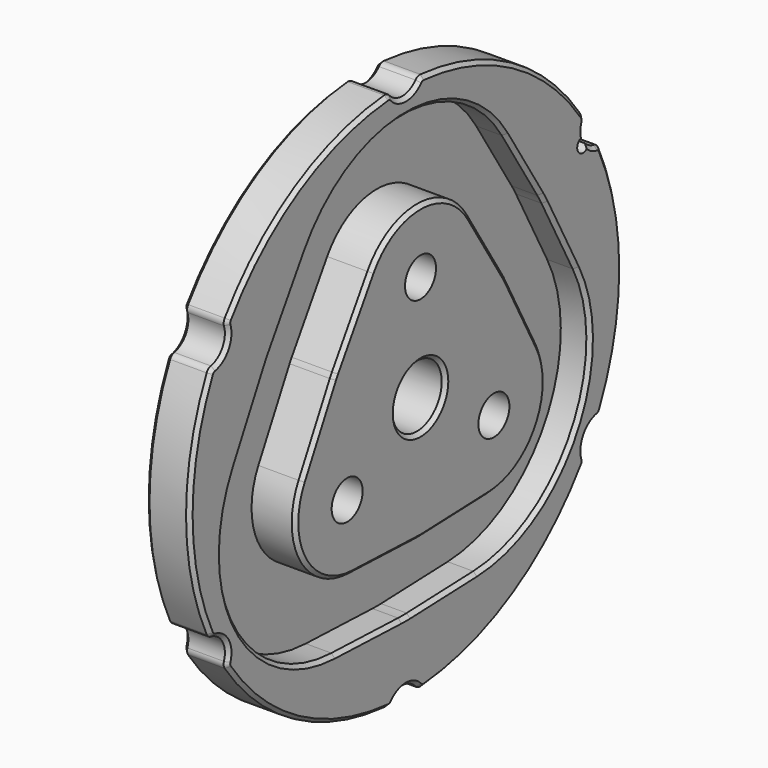
from build123d import *

# Parameters (mm, degrees)
F0_R     = 2.65
F0_R_2   = 4.25
F1_DEPTH = 6
F2_DEPTH = 4
F3_DEPTH = 2
F4_SIZE  = 0.5
F5_SIZE2 = 2.3
F5_SIZE  = 5


# Not quite as in the source:
# - two fillets or chamfers of one size are made in one step


with BuildPart() as f1:
    # F0 (on Right) → F1 (new body)
    with BuildSketch(Plane.YZ):
        with BuildLine():
            ThreePointArc((-2.2515407231, 36.53242851), (-2.6294191421, 36.8013801393), (-3.0879953604, 36.8709138028))
            ThreePointArc((-3.0879953604, 36.8709138028), (-18.5, 32.04293994), (-30.3871503338, 21.1097393303))
            ThreePointArc((-30.3871503338, 21.1097393303), (-30.5562205239, 20.6778338439), (-30.5122407901, 20.2161057189))
            ThreePointArc((-30.5122407901, 20.2161057189), (-30.7524645978, 17.7549437138), (-32.7637815132, 16.3163227911))
            ThreePointArc((-32.7637815132, 16.3163227911), (-33.185639666, 16.1235462954), (-33.4751456942, 15.7611744725))
            ThreePointArc((-33.4751456942, 15.7611744725), (-37, 0), (-33.4751456942, -15.7611744725))
            ThreePointArc((-33.4751456942, -15.7611744725), (-33.185639666, -16.1235462954), (-32.7637815132, -16.3163227911))
            ThreePointArc((-32.7637815132, -16.3163227911), (-30.7524645978, -17.7549437138), (-30.5122407901, -20.2161057189))
            ThreePointArc((-30.5122407901, -20.2161057189), (-30.5562205239, -20.6778338439), (-30.3871503338, -21.1097393303))
            ThreePointArc((-30.3871503338, -21.1097393303), (-18.5, -32.04293994), (-3.0879953604, -36.8709138028))
            ThreePointArc((-3.0879953604, -36.8709138028), (-2.6294191421, -36.8013801393), (-2.2515407231, -36.53242851))
            ThreePointArc((-2.2515407231, -36.53242851), (0, -35.5098874275), (2.2515407231, -36.53242851))
            ThreePointArc((2.2515407231, -36.53242851), (2.6294191421, -36.8013801393), (3.0879953604, -36.8709138028))
            ThreePointArc((3.0879953604, -36.8709138028), (18.5, -32.04293994), (30.3871503338, -21.1097393303))
            ThreePointArc((30.3871503338, -21.1097393303), (30.5562205239, -20.6778338439), (30.5122407901, -20.2161057189))
            ThreePointArc((30.5122407901, -20.2161057189), (30.7524645978, -17.7549437138), (32.7637815132, -16.3163227911))
            ThreePointArc((32.7637815132, -16.3163227911), (33.185639666, -16.1235462954), (33.4751456942, -15.7611744725))
            ThreePointArc((33.4751456942, -15.7611744725), (37, 0), (33.4751456942, 15.7611744725))
            ThreePointArc((33.4751456942, 15.7611744725), (33.185639666, 16.1235462954), (32.7637815132, 16.3163227911))
            ThreePointArc((32.7637815132, 16.3163227911), (31.941237039, 16.6082774884), (31.2380455813, 17.1253255822))
            ThreePointArc((31.2380455813, 17.1253255822), (29.4448637287, 17), (30.449989793, 18.4902782469))
            ThreePointArc((30.449989793, 18.4902782469), (30.3538087376, 19.3577839598), (30.5122407901, 20.2161057189))
            ThreePointArc((30.5122407901, 20.2161057189), (30.5562205239, 20.6778338439), (30.3871503338, 21.1097393303))
            ThreePointArc((30.3871503338, 21.1097393303), (18.5, 32.04293994), (3.0879953604, 36.8709138028))
            ThreePointArc((3.0879953604, 36.8709138028), (2.6294191421, 36.8013801393), (2.2515407231, 36.53242851))
            ThreePointArc((2.2515407231, 36.53242851), (0, 35.5098874275), (-2.2515407231, 36.53242851))
        make_face()
        with BuildLine():
            Line((-23.0952370323, 14.180454946), (-17.0328632471, 23.8484731203))
            ThreePointArc((-17.0328632471, 23.8484731203), (0.0002590164, 33.2703478915), (17.0295377344, 23.8415279974))
            Line((17.0295377344, 23.8415279974), (23.0899184639, 14.167925942))
            ThreePointArc((23.0899184639, 14.167925942), (23.4636524397, 13.5467460522), (23.8147430167, 12.9124929901))
            Line((23.8147430167, 12.9124929901), (29.162137778, 2.827248294))
            ThreePointArc((29.162137778, 2.827248294), (28.813095975, -16.6349496309), (12.1369519401, -26.6751288313))
            Line((12.1369519401, -26.6751288313), (0.7330157043, -27.0912894495))
            ThreePointArc((0.7330157043, -27.0912894495), (0, -27.1046598669), (-0.7330157043, -27.0912894495))
            Line((-0.7330157043, -27.0912894495), (-12.1441739659, -26.6748652799))
            ThreePointArc((-12.1441739659, -26.6748652799), (-28.8182692269, -16.6382354957), (-29.1731979579, 2.8202694775))
            Line((-29.1731979579, 2.8202694775), (-23.8282527367, 12.9108345034))
            ThreePointArc((-23.8282527367, 12.9108345034), (-23.4733240056, 13.5523299334), (-23.0952370323, 14.180454946))
        make_face(mode=Mode.SUBTRACT)
        with BuildLine():
            ThreePointArc((17.0295377344, 23.8415279974), (0.0002590164, 33.2703478915), (-17.0328632471, 23.8484731203))
            Line((-17.0328632471, 23.8484731203), (-23.0952370323, 14.180454946))
            ThreePointArc((-23.0952370323, 14.180454946), (-23.4733240056, 13.5523299334), (-23.8282527367, 12.9108345034))
            Line((-23.8282527367, 12.9108345034), (-29.1731979579, 2.8202694775))
            ThreePointArc((-29.1731979579, 2.8202694775), (-28.8182692269, -16.6382354957), (-12.1441739659, -26.6748652799))
            Line((-12.1441739659, -26.6748652799), (-0.7330157043, -27.0912894495))
            ThreePointArc((-0.7330157043, -27.0912894495), (0, -27.1046598669), (0.7330157043, -27.0912894495))
            Line((0.7330157043, -27.0912894495), (12.1369519401, -26.6751288313))
            ThreePointArc((12.1369519401, -26.6751288313), (28.813095975, -16.6349496309), (29.162137778, 2.827248294))
            Line((29.162137778, 2.827248294), (23.8147430167, 12.9124929901))
            ThreePointArc((23.8147430167, 12.9124929901), (23.4636524397, 13.5467460522), (23.0899184639, 14.167925942))
            Line((23.0899184639, 14.167925942), (17.0295377344, 23.8415279974))
        make_face()
        with BuildLine():
            Line((-14.5383641102, 8.8148297318), (-8.4759903249, 18.482847906))
            ThreePointArc((-8.4759903249, 18.482847906), (-0.0018003141, 23.1703476982), (8.4704774851, 18.4793926211))
            Line((8.4704774851, 18.4793926211), (14.5308582146, 8.8057905657))
            ThreePointArc((14.5308582146, 8.8057905657), (14.7167955123, 8.4967458506), (14.8914674376, 8.1811970698))
            Line((14.8914674376, 8.1811970698), (20.2388621989, -1.9040476263))
            ThreePointArc((20.2388621989, -1.9040476263), (20.0652095641, -11.5867329668), (11.7686206585, -16.5818468966))
            Line((11.7686206585, -16.5818468966), (0.3646844227, -16.9980075148))
            ThreePointArc((0.3646844227, -16.9980075148), (0, -17.0046594636), (-0.3646844227, -16.9980075148))
            Line((-0.3646844227, -16.9980075148), (-11.7758426843, -16.5815833453))
            ThreePointArc((-11.7758426843, -16.5815833453), (-20.0714122995, -11.5882352941), (-20.2479937541, -1.9073872429))
            Line((-20.2479937541, -1.9073872429), (-14.9030485329, 8.183177783))
            ThreePointArc((-14.9030485329, 8.183177783), (-14.7264670782, 8.5023297318), (-14.5383641102, 8.8148297318))
        make_face(mode=Mode.SUBTRACT)
        with BuildLine():
            ThreePointArc((8.4704774851, 18.4793926211), (-0.0018003141, 23.1703476982), (-8.4759903249, 18.482847906))
            Line((-8.4759903249, 18.482847906), (-14.5383641102, 8.8148297318))
            ThreePointArc((-14.5383641102, 8.8148297318), (-14.7264670782, 8.5023297318), (-14.9030485329, 8.183177783))
            Line((-14.9030485329, 8.183177783), (-20.2479937541, -1.9073872429))
            ThreePointArc((-20.2479937541, -1.9073872429), (-20.0714122995, -11.5882352941), (-11.7758426843, -16.5815833453))
            Line((-11.7758426843, -16.5815833453), (-0.3646844227, -16.9980075148))
            ThreePointArc((-0.3646844227, -16.9980075148), (0, -17.0046594636), (0.3646844227, -16.9980075148))
            Line((0.3646844227, -16.9980075148), (11.7686206585, -16.5818468966))
            ThreePointArc((11.7686206585, -16.5818468966), (20.0652095641, -11.5867329668), (20.2388621989, -1.9040476263))
            Line((20.2388621989, -1.9040476263), (14.8914674376, 8.1811970698))
            ThreePointArc((14.8914674376, 8.1811970698), (14.7167955123, 8.4967458506), (14.5308582146, 8.8057905657))
            Line((14.5308582146, 8.8057905657), (8.4704774851, 18.4793926211))
        make_face()
        with Locations((-12.5573683549, -7.25)):
            Circle(F0_R, mode=Mode.SUBTRACT)
        with Locations((12.5573683549, -7.25)):
            Circle(F0_R, mode=Mode.SUBTRACT)
        Circle(F0_R_2, mode=Mode.SUBTRACT)
        with Locations((0, 14.5)):
            Circle(F0_R, mode=Mode.SUBTRACT)
    extrude(amount=-F1_DEPTH)

    # F0 (on Right) → F2 (cut)
    with BuildSketch(Plane.YZ):
        with BuildLine():
            ThreePointArc((17.0295377344, 23.8415279974), (0.0002590164, 33.2703478915), (-17.0328632471, 23.8484731203))
            Line((-17.0328632471, 23.8484731203), (-23.0952370323, 14.180454946))
            ThreePointArc((-23.0952370323, 14.180454946), (-23.4733240056, 13.5523299334), (-23.8282527367, 12.9108345034))
            Line((-23.8282527367, 12.9108345034), (-29.1731979579, 2.8202694775))
            ThreePointArc((-29.1731979579, 2.8202694775), (-28.8182692269, -16.6382354957), (-12.1441739659, -26.6748652799))
            Line((-12.1441739659, -26.6748652799), (-0.7330157043, -27.0912894495))
            ThreePointArc((-0.7330157043, -27.0912894495), (0, -27.1046598669), (0.7330157043, -27.0912894495))
            Line((0.7330157043, -27.0912894495), (12.1369519401, -26.6751288313))
            ThreePointArc((12.1369519401, -26.6751288313), (28.813095975, -16.6349496309), (29.162137778, 2.827248294))
            Line((29.162137778, 2.827248294), (23.8147430167, 12.9124929901))
            ThreePointArc((23.8147430167, 12.9124929901), (23.4636524397, 13.5467460522), (23.0899184639, 14.167925942))
            Line((23.0899184639, 14.167925942), (17.0295377344, 23.8415279974))
        make_face()
        with BuildLine():
            Line((-14.5383641102, 8.8148297318), (-8.4759903249, 18.482847906))
            ThreePointArc((-8.4759903249, 18.482847906), (-0.0018003141, 23.1703476982), (8.4704774851, 18.4793926211))
            Line((8.4704774851, 18.4793926211), (14.5308582146, 8.8057905657))
            ThreePointArc((14.5308582146, 8.8057905657), (14.7167955123, 8.4967458506), (14.8914674376, 8.1811970698))
            Line((14.8914674376, 8.1811970698), (20.2388621989, -1.9040476263))
            ThreePointArc((20.2388621989, -1.9040476263), (20.0652095641, -11.5867329668), (11.7686206585, -16.5818468966))
            Line((11.7686206585, -16.5818468966), (0.3646844227, -16.9980075148))
            ThreePointArc((0.3646844227, -16.9980075148), (0, -17.0046594636), (-0.3646844227, -16.9980075148))
            Line((-0.3646844227, -16.9980075148), (-11.7758426843, -16.5815833453))
            ThreePointArc((-11.7758426843, -16.5815833453), (-20.0714122995, -11.5882352941), (-20.2479937541, -1.9073872429))
            Line((-20.2479937541, -1.9073872429), (-14.9030485329, 8.183177783))
            ThreePointArc((-14.9030485329, 8.183177783), (-14.7264670782, 8.5023297318), (-14.5383641102, 8.8148297318))
        make_face(mode=Mode.SUBTRACT)
    extrude(amount=-F2_DEPTH, mode=Mode.SUBTRACT)

    # F3 (add): a face of the model
    f3_faces = [f1.faces().sort_by_distance(p)[0] for p in [
        (0, -11.0097556238, 13.3369283968),
    ]]
    extrude(f3_faces, amount=F3_DEPTH)

    # F4
    f4_edges = [f1.edges().sort_by_distance(p)[0] for p in [
        (-6, 18.5, -32.04294),
        (0, 18.5, -32.04294),
        (0, 28.813096, -16.63495),
        (2, 20.06521, -11.586733),
        (2, -4.25, 0),
        (0, 30.556221, 20.677834),
        (-6, 30.556221, 20.677834),
        (0, 30.353809, 19.357784),
        (-6, 30.353809, 19.357784),
        (0, 18.5, 32.04294),
        (-6, 18.5, 32.04294),
        (0, 2.629419, 36.80138),
        (0, 31.941237, 16.608277),
        (0, 0, 35.509887),
        (0, 33.18564, 16.123546),
        (0, -2.629419, 36.80138),
        (0, 37, 0),
        (0, -18.5, 32.04294),
        (0, 33.18564, -16.123546),
        (0, -30.556221, 20.677834),
        (0, 30.752465, -17.754944),
        (0, -30.752465, 17.754944),
        (0, 30.556221, -20.677834),
        (0, -33.18564, 16.123546),
        (0, -37, 0),
        (0, 2.629419, -36.80138),
        (0, -33.18564, -16.123546),
        (0, 0, -35.509887),
        (0, -30.752465, -17.754944),
        (0, -2.629419, -36.80138),
        (0, -30.556221, -20.677834),
        (0, -18.5, -32.04294),
        (0, 23.463652, 13.546746),
        (0, 20.059728, 19.004727),
        (0, 0.000259, 33.270348),
        (0, -20.06405, 19.014464),
        (0, -23.473324, 13.55233),
        (0, -26.500725, 7.865552),
        (0, -28.818269, -16.638235),
        (0, -6.438595, -26.883077),
        (0, 0, -27.10466),
        (0, 6.434984, -26.883209),
        (0, 26.48844, 7.869871),
        (-6, 2.629419, 36.80138),
        (-6, 0, 35.509887),
        (-6, -2.629419, 36.80138),
        (-6, -18.5, 32.04294),
        (-6, -30.556221, 20.677834),
        (-6, -30.752465, 17.754944),
        (-6, -33.18564, 16.123546),
        (-6, -37, 0),
        (-6, -33.18564, -16.123546),
        (-6, -30.752465, -17.754944),
        (-6, -30.556221, -20.677834),
        (-6, -18.5, -32.04294),
        (-6, -2.629419, -36.80138),
        (-6, 0, -35.509887),
        (-6, 2.629419, -36.80138),
        (-6, 30.556221, -20.677834),
        (-6, 30.752465, -17.754944),
        (-6, 33.18564, -16.123546),
        (-6, 37, 0),
        (-6, 33.18564, 16.123546),
        (-6, 31.941237, 16.608277),
        (-6, -4.25, 0),
        (2, -11.507177, 13.648839),
        (2, -0.0018, 23.170348),
        (2, 11.500668, 13.642592),
        (2, 14.716796, 8.496746),
        (2, 17.565165, 3.138575),
        (2, 6.066653, -16.789927),
        (2, 0, -17.004659),
        (2, -6.070264, -16.789795),
        (2, -20.071412, -11.588235),
        (2, -17.575521, 3.137895),
        (2, -14.726467, 8.50233),
    ]]
    chamfer(f4_edges, length=F4_SIZE)

    # F5
    f5_edges = [f1.edges().sort_by_distance(p)[0] for p in [
        (-6, -2.65, 14.5),
        (-6, -15.207368, -7.25),
        (-6, 9.907368, -7.25),
    ]]
    f5_side = f1.faces().sort_by_distance((-6, 28.552337, 16.484699))[0]
    chamfer(f5_edges, length=F5_SIZE, length2=F5_SIZE2, reference=f5_side)


solid = f1.part
